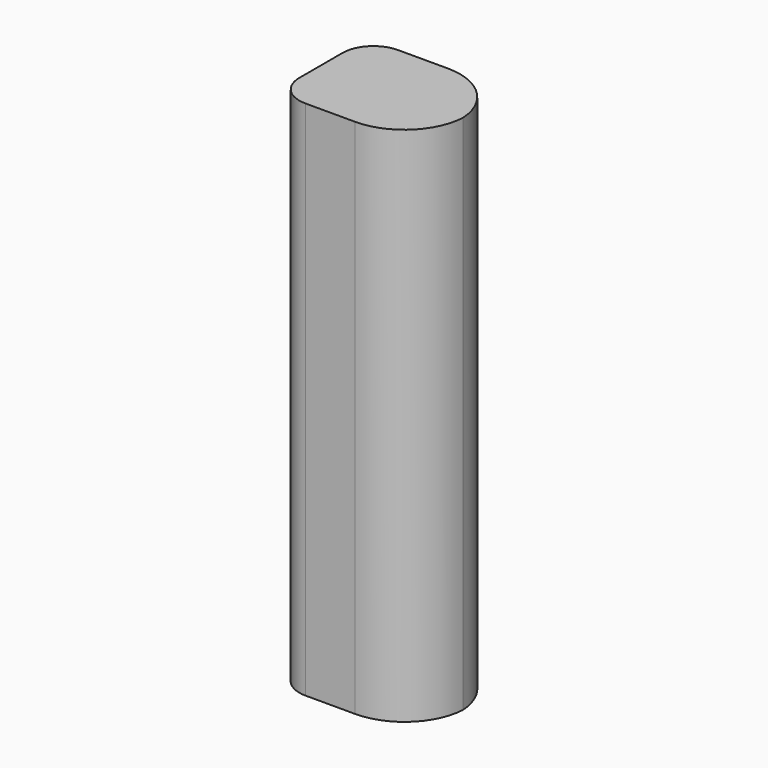
from build123d import *

# Parameters (mm, degrees)
F1_DEPTH    = 9.525
F0_W        = 23.402531108
F0_H        = 85.8396906406
F3_T1_DEPTH = 136.6396906406
F4_R        = 5.08


# Not quite as in the source:
# - a fillet or chamfer that OpenCascade refuses, or shapes differently, is made with other operations: its cross-section is extruded or revolved along the edge and cut away or added


with BuildPart() as f1:
    # F0 (on Front) → F1 (new body, symmetric)
    with BuildSketch(Plane.XZ):
        Polygon((-2.3270829115, -113.9840111136), (-12.9329506308, -113.9840111136), (-12.9329506308, -186.3234937191), (-2.3270829115, -199.3203783987), (8.2787848078, -186.3234937191), (8.2787848078, -113.9840111136), align=None)
    extrude(amount=F1_DEPTH, both=True)


with BuildPart() as f1b:
    # F0 (on Front) → F1, piece 2 (new body, symmetric)
    with BuildSketch(Plane.XZ):
        with Locations((-1.2316850768, -52.651762031)):
            Rectangle(F0_W, F0_H)
    extrude(amount=F1_DEPTH, both=True)

    # F3: fillet of radius 10.16 on 2 edges, made by hand

    # F3_s2 → F3_t1 (cut)
    with BuildSketch(Plane.XY.offset(-120.9716073513)):
        with BuildLine():
            ThreePointArc((0.3095804772, -9.525), (7.4937853741, -6.5492048969), (10.4695804772, 0.635))
            Line((10.4695804772, 0.635), (10.4695804772, -9.525))
            Line((10.4695804772, -9.525), (0.3095804772, -9.525))
        make_face()
        with BuildLine():
            ThreePointArc((10.4695804772, -0.635), (7.4937853741, 6.5492048969), (0.3095804772, 9.525))
            Line((0.3095804772, 9.525), (10.4695804772, 9.525))
            Line((10.4695804772, 9.525), (10.4695804772, -0.635))
        make_face()
    extrude(amount=F3_T1_DEPTH, mode=Mode.SUBTRACT)

    # F4
    f4_edges = [f1b.edges().sort_by_distance(p)[0] for p in [
        (-12.932951, 9.525, -52.651762),
        (-12.932951, -9.525, -52.651762),
    ]]
    fillet(f4_edges, radius=F4_R)


solid = f1b.part
